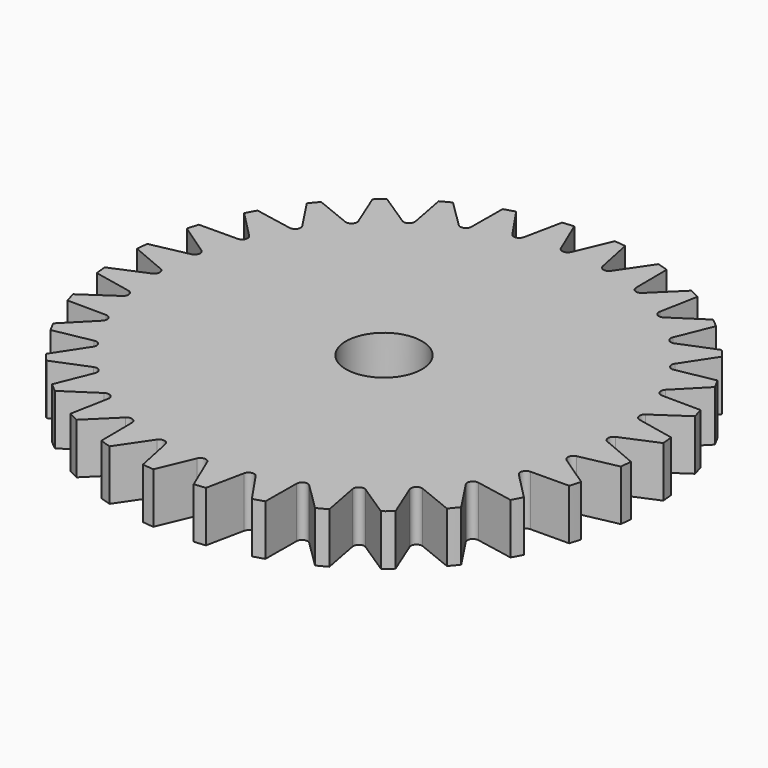
from build123d import *

# Parameters (mm, degrees)
F0_R            = 21.158401666
F0_R_2          = 3.048
F1_DEPTH        = 4.064
F3_DEPTH        = 4.064
F3_COPIES_COUNT = 32


# Not quite as in the source:
# - a pattern or mirror of a feature is missing from the dataset's text; its kind, count and spacing are read off the source's solid


with BuildPart() as f1:
    # F0 (on Top) → F1 (new body)
    with BuildSketch(Plane.XY):
        Circle(F0_R)
        Circle(F0_R_2, mode=Mode.SUBTRACT)
    extrude(amount=F1_DEPTH)

    # F2 (on face) → F3 (cut, through all)
    with BuildSketch(Plane.XY.offset(4.064)):
        with BuildLine():
            Line((-0.4109729921, -18.2450008044), (-1.6185707702, -21.0964022933))
            ThreePointArc((-1.6185707702, -21.0964022933), (0, -21.158401666), (1.6185707702, -21.0964022933))
            Line((1.6185707702, -21.0964022933), (0.4109729921, -18.2450008044))
            ThreePointArc((0.4109729921, -18.2450008044), (0, -17.9727420469), (-0.4109729921, -18.2450008044))
        make_face()
    f3 = extrude(amount=-F3_DEPTH, mode=Mode.SUBTRACT)

    # F3_copies: F3 ×32 about axis
    f3_copies_axis = Axis((0, 0, 0), (0, 0, 1))
    for i in range(1, F3_COPIES_COUNT):
        add(f3.rotate(f3_copies_axis, i * 360 / F3_COPIES_COUNT), mode=Mode.SUBTRACT)


solid = f1.part
